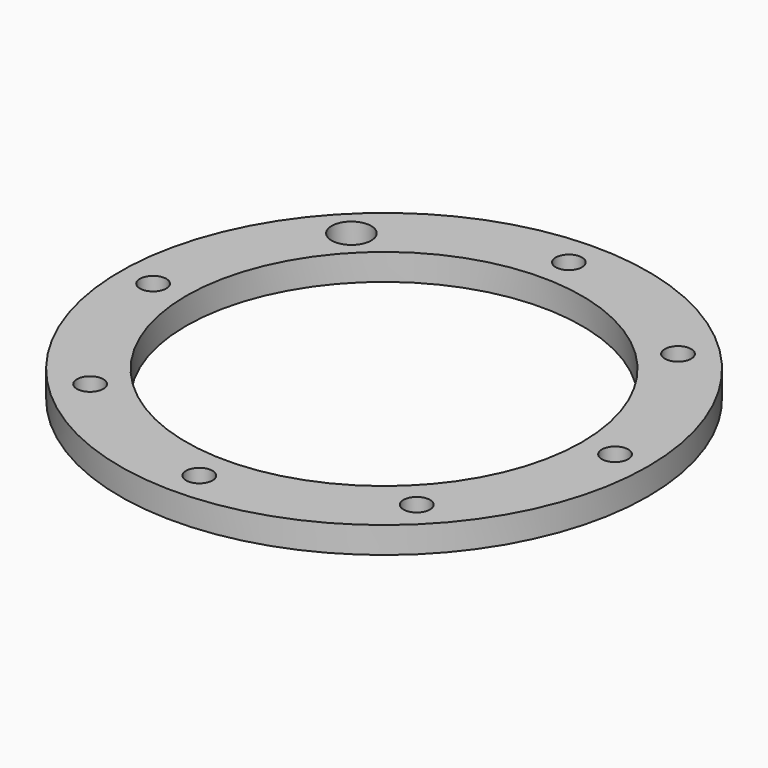
from build123d import *

# Parameters (mm, degrees)
F0_R            = 100
F1_DEPTH        = 10
F2_R            = 75
F3_DEPTH        = 10.001
F4_R            = 5
F5_DEPTH        = 10.001
F5_COPIES_COUNT = 7
F5_COPIES_ANGLE = 270
F8_R            = 7.5
F9_DEPTH        = 10.001


# Not quite as in the source:
# - a pattern or mirror of a feature is missing from the dataset's text; its kind, count and spacing are read off the source's solid


with BuildPart() as f1:
    # F0 (on Top) → F1 (new body)
    with BuildSketch(Plane.XY):
        Circle(F0_R)
    extrude(amount=F1_DEPTH)

    # F2 (on face) → F3 (cut, through all)
    with BuildSketch(Plane.XY.offset(10)):
        Circle(F2_R)
    extrude(amount=-F3_DEPTH, mode=Mode.SUBTRACT)

    # F4 (on face) → F5 (cut, through all)
    with BuildSketch(Plane.XY.offset(10)):
        with Locations((-87.5, 0)):
            Circle(F4_R)
    f5 = extrude(amount=-F5_DEPTH, mode=Mode.SUBTRACT)

    # F5_copies: F5 ×7 about axis
    f5_copies_axis = Axis((0, 0, 0), (0, 0, 1))
    for i in range(1, F5_COPIES_COUNT):
        add(f5.rotate(f5_copies_axis, i * F5_COPIES_ANGLE / (F5_COPIES_COUNT - 1)), mode=Mode.SUBTRACT)

    # F8 (on face) → F9 (cut, through all)
    with BuildSketch(Plane.XY.offset(10)):
        with Locations((-61.8718433538, 61.8718433538)):
            Circle(F8_R)
    extrude(amount=-F9_DEPTH, mode=Mode.SUBTRACT)


solid = f1.part
